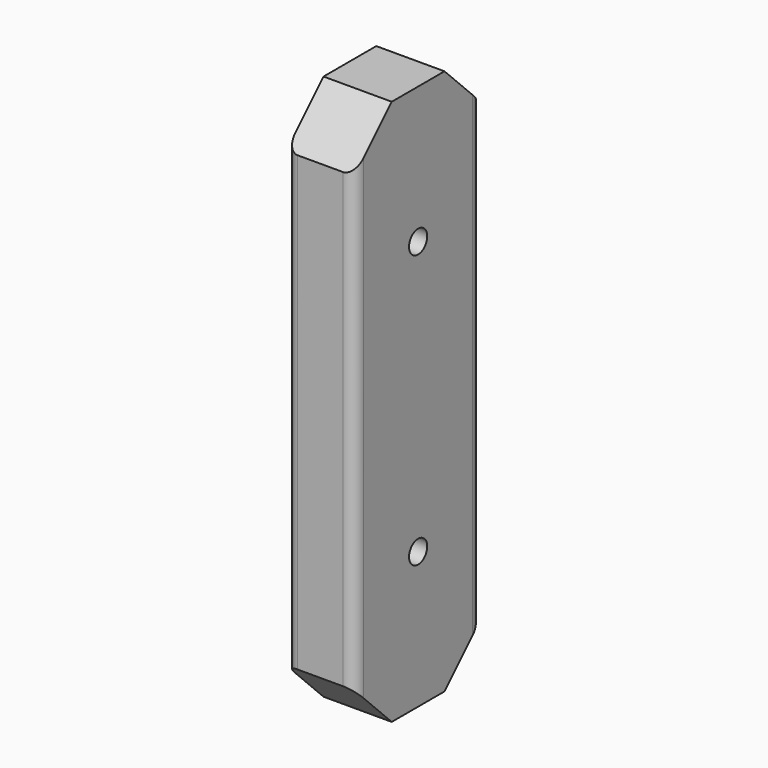
from build123d import *

# Parameters (mm, degrees)
F1_DEPTH = 304.8
F3_DEPTH = 50.8
F4_D     = 12.7


with BuildPart() as f1:
    # F0 (on Top) → F1 (new body)
    with BuildSketch(Plane.XY):
        with BuildLine():
            Line((-12.7, -44.45), (12.7, -44.45))
            ThreePointArc((12.7, -44.45), (17.1901280605, -42.5901280605), (19.05, -38.1))
            Line((19.05, -38.1), (19.05, 38.1))
            ThreePointArc((19.05, 38.1), (17.1901280605, 42.5901280605), (12.7, 44.45))
            Line((12.7, 44.45), (-12.7, 44.45))
            ThreePointArc((-12.7, 44.45), (-17.1901280605, 42.5901280605), (-19.05, 38.1))
            Line((-19.05, 38.1), (-19.05, -38.1))
            ThreePointArc((-19.05, -38.1), (-17.1901280605, -42.5901280605), (-12.7, -44.45))
        make_face()
    extrude(amount=F1_DEPTH)

    # F2 (on face) → F3 (cut)
    with BuildSketch(Plane(origin=(-19.05, 0, 0), x_dir=(0, -1, 0), z_dir=(-1, 0, 0))):
        Polygon((-38.1, 304.8), (-44.45, 304.8), (-44.45, 278.7617928475), (-38.1, 285.1117928475), align=None)
        Polygon((-18.4117928475, 304.8), (-38.1, 304.8), (-38.1, 285.1117928475), align=None)
        Polygon((-38.1, 19.6882071525), (-44.45, 26.0382071525), (-44.45, 0), (-38.1, 0), align=None)
        Polygon((-18.4117928475, 0), (-38.1, 19.6882071525), (-38.1, 0), align=None)
        Polygon((38.1, 304.8), (18.4117928475, 304.8), (38.1, 285.1117928475), align=None)
        Polygon((44.45, 304.8), (38.1, 304.8), (38.1, 285.1117928475), (44.45, 278.7617928475), align=None)
        Polygon((38.1, 19.6882071525), (18.4117928475, 0), (38.1, 0), align=None)
        Polygon((44.45, 26.0382071525), (38.1, 19.6882071525), (38.1, 0), (44.45, 0), align=None)
    extrude(amount=-F3_DEPTH, mode=Mode.SUBTRACT)

    # F4 (through all)
    with Locations(Plane(origin=(-19.05, 0, 0), x_dir=(0, -1, 0), z_dir=(-1, 0, 0))):
        with Locations((0, 76.2), (0, 228.6)):
            Hole(F4_D / 2)


solid = f1.part
